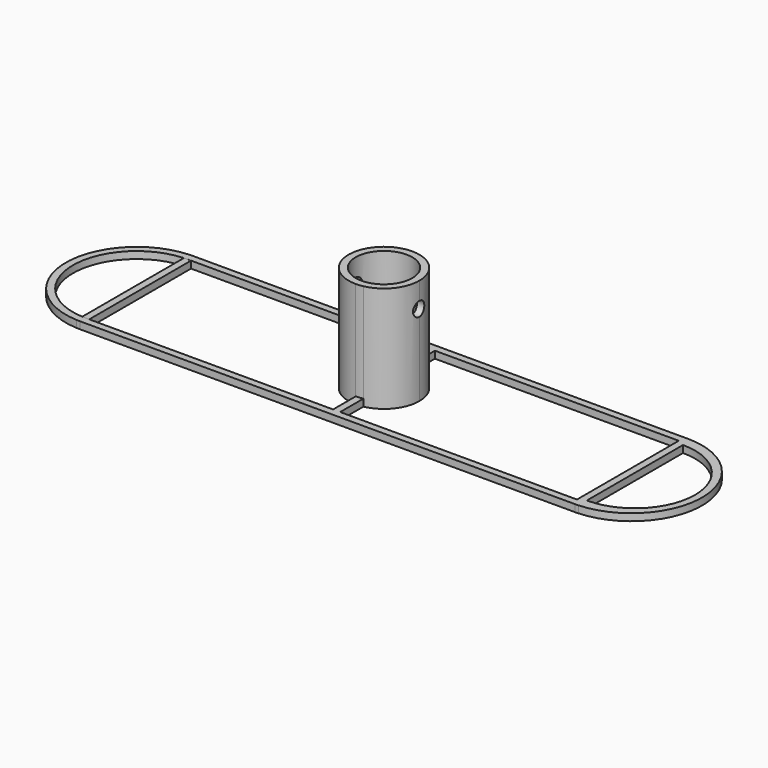
from build123d import *

# Parameters (mm, degrees)
F0_W     = 1
F0_H     = 1
F0_W_2   = 34.5
F0_H_2   = 3
F0_W_3   = 33.5
F1_DEPTH = 1
F0_R     = 4
F2_DEPTH = 15
F3_R     = 1
F4_DEPTH = 12.5


with BuildPart() as f1:
    # F0 (on Top) → F1 (new body)
    with BuildSketch(Plane.XY):
        with BuildLine():
            Line((-1, 10), (-35, 10))
            ThreePointArc((-35, 10), (-35.2500782106, 9.9968725554), (-35.5, 9.9874921777))
            Line((-35.5, 9.9874921777), (-34.5, 9.9874921777))
            Line((-34.5, 9.9874921777), (-34.5, 9))
            Line((-34.5, 9), (-1, 9))
            Line((-1, 9), (-1, 10))
        make_face()
        with Locations((-0.5, 9.5)):
            Rectangle(F0_W, F0_H)
        with BuildLine():
            Line((-35.5, 9), (-35.5, 9.9874921777))
            ThreePointArc((-35.5, 9.9874921777), (-45, 0), (-35.5, -9.9874921777))
            Line((-35.5, -9.9874921777), (-35.5, -9))
            Line((-35.5, -9), (-35.5, -8.9861003778))
            ThreePointArc((-35.5, -8.9861003778), (-44, 0), (-35.5, 8.9861003778))
            Line((-35.5, 8.9861003778), (-35.5, 9))
        make_face()
        Polygon((-34.5, 9.9874921777), (-35.5, 9.9874921777), (-35.5, 9), (-35, 9), (-34.5, 9), align=None)
        with Locations((17.25, 9.5)):
            Rectangle(F0_W_2, F0_H)
        with Locations((-0.5, 7.5)):
            Rectangle(F0_W, F0_H_2)
        with BuildLine():
            Line((-34.5, -9.9874921777), (-35.5, -9.9874921777))
            ThreePointArc((-35.5, -9.9874921777), (-35.2500782106, -9.9968725554), (-35, -10))
            Line((-35, -10), (0, -10))
            Line((0, -10), (0, -9))
            Line((0, -9), (-34.5, -9))
            Line((-34.5, -9), (-34.5, -9.9874921777))
        make_face()
        Polygon((-35.5, -9), (-35.5, -9.9874921777), (-34.5, -9.9874921777), (-34.5, -9), (-35, -9), align=None)
        with BuildLine():
            Line((35, 10), (34.5, 10))
            Line((34.5, 10), (34.5, 9))
            Line((34.5, 9), (35.5, 9))
            Line((35.5, 9), (35.5, 9.9874921777))
            ThreePointArc((35.5, 9.9874921777), (35.2500782106, 9.9968725554), (35, 10))
        make_face()
        with BuildLine():
            Line((0, 6), (-1, 6))
            Line((-1, 6), (-1, 4.8989794856))
            ThreePointArc((-1, 4.8989794856), (-0.50254481, 4.974680765), (0, 5))
            Line((0, 5), (0, 6))
        make_face()
        with BuildLine():
            Line((35.5, 9), (34.5, 9))
            Line((34.5, 9), (34.5, 8.4409715081))
            ThreePointArc((34.5, 8.4409715081), (34.9991296668, 8.4852300446), (35.5, 8.5))
            Line((35.5, 8.5), (35.5, 9))
        make_face()
        with Locations((0.5, -9.5)):
            Rectangle(F0_W, F0_H)
        with BuildLine():
            ThreePointArc((35.5, -9.9874921777), (45, 0), (35.5, 9.9874921777))
            Line((35.5, 9.9874921777), (35.5, 9))
            Line((35.5, 9), (35.5, 8.5))
            ThreePointArc((35.5, 8.5), (44, 0), (35.5, -8.5))
            Line((35.5, -8.5), (35.5, -9))
            Line((35.5, -9), (35.5, -9.9874921777))
        make_face()
        with BuildLine():
            ThreePointArc((35.5, 8.5), (34.9991296668, 8.4852300446), (34.5, 8.4409715081))
            Line((34.5, 8.4409715081), (34.5, -8.4409715081))
            ThreePointArc((34.5, -8.4409715081), (34.9991296668, -8.4852300446), (35.5, -8.5))
            Line((35.5, -8.5), (35.5, 8.5))
        make_face()
        with BuildLine():
            ThreePointArc((1, -4.8989794856), (0.50254481, -4.974680765), (0, -5))
            Line((0, -5), (0, -6))
            Line((0, -6), (1, -6))
            Line((1, -6), (1, -4.8989794856))
        make_face()
        with Locations((17.75, -9.5)):
            Rectangle(F0_W_3, F0_H)
        with Locations((0.5, -7.5)):
            Rectangle(F0_W, F0_H_2)
        with BuildLine():
            ThreePointArc((35, -10), (35.2500782106, -9.9968725554), (35.5, -9.9874921777))
            Line((35.5, -9.9874921777), (35.5, -9))
            Line((35.5, -9), (34.5, -9))
            Line((34.5, -9), (34.5, -10))
            Line((34.5, -10), (35, -10))
        make_face()
        with BuildLine():
            ThreePointArc((35.5, -8.5), (34.9991296668, -8.4852300446), (34.5, -8.4409715081))
            Line((34.5, -8.4409715081), (34.5, -9))
            Line((34.5, -9), (35.5, -9))
            Line((35.5, -9), (35.5, -8.5))
        make_face()
    extrude(amount=F1_DEPTH)

    # F0 (on Top) → F2 (join)
    with BuildSketch(Plane.XY):
        with BuildLine():
            ThreePointArc((0, 5), (-0.50254481, 4.974680765), (-1, 4.8989794856))
            ThreePointArc((-1, 4.8989794856), (-4.974680765, -0.50254481), (0, -5))
            ThreePointArc((0, -5), (0.50254481, -4.974680765), (1, -4.8989794856))
            ThreePointArc((1, -4.8989794856), (3.8729833462, -3.1622776602), (5, 0))
            ThreePointArc((5, 0), (3.5355339059, 3.5355339059), (0, 5))
        make_face()
        Circle(F0_R, mode=Mode.SUBTRACT)
    extrude(amount=F2_DEPTH)

    # F3 (on Right) → F4 (cut, symmetric)
    with BuildSketch(Plane.YZ):
        with Locations((0, 11.4876687593)):
            Circle(F3_R)
    extrude(amount=F4_DEPTH, both=True, mode=Mode.SUBTRACT)


with BuildPart() as f1b:
    # F0 (on Top) → F1, piece 2 (new body)
    with BuildSketch(Plane.XY):
        with BuildLine():
            ThreePointArc((-35, 9), (-35.2500965811, 8.9965244234), (-35.5, 8.9861003778))
            Line((-35.5, 8.9861003778), (-35.5, -8.9861003778))
            ThreePointArc((-35.5, -8.9861003778), (-35.2500965811, -8.9965244234), (-35, -9))
            ThreePointArc((-35, -9), (-34.7499034189, -8.9965244234), (-34.5, -8.9861003778))
            Line((-34.5, -8.9861003778), (-34.5, 8.9861003778))
            ThreePointArc((-34.5, 8.9861003778), (-34.7499034189, 8.9965244234), (-35, 9))
        make_face()
    extrude(amount=F1_DEPTH)


solid = Compound([f1.part, f1b.part])
